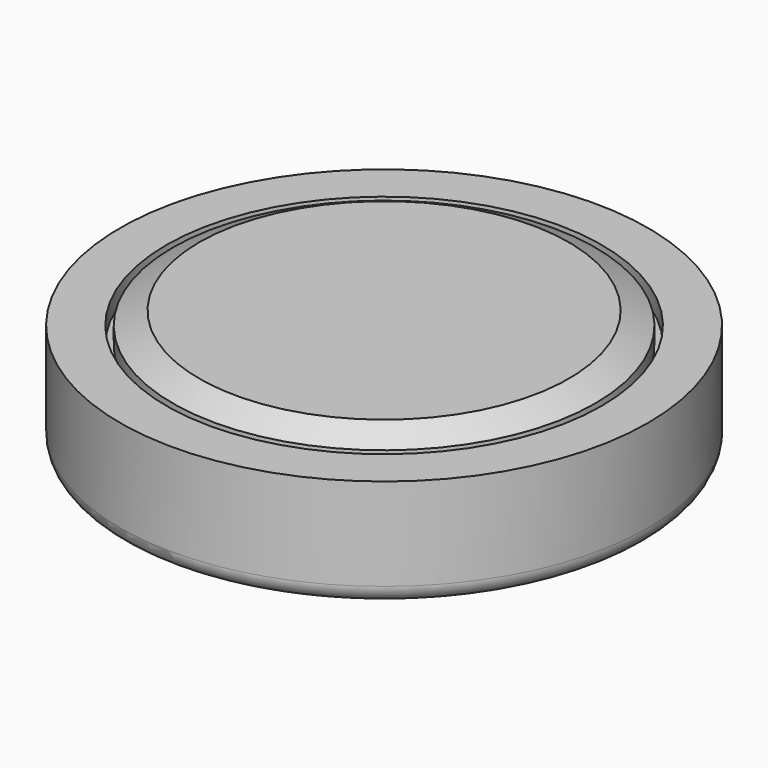
from build123d import *

# Parameters (mm, degrees)
F0_R      = 1.25
F1_DEPTH  = 3
F3_DEPTH  = 6
F4_R      = 1.2192
F5_DEPTH  = 7
F4_R_2    = 2
F4_R_3    = 0.9271
F7_R      = 24
F7_R_2    = 22
F7_R_3    = 21
F8_DEPTH  = 1.5
F9_DEPTH  = 2
F12_DEPTH = 2
F14_R     = 30
F14_R_2   = 24.75
F14_R_3   = 22.75
F14_R_4   = 2.75
F14_R_5   = 0.75
F14_R_6   = 1.875
F15_DEPTH = 2
F16_DEPTH = 1.5
F18_DEPTH = 8.5
F19_DEPTH = 10.5
F20_R     = 1.99999


# Not quite as in the source:
# - a fillet or chamfer that OpenCascade refuses, or shapes differently, is made with other operations: its cross-section is extruded or revolved along the edge and cut away or added
# - a fillet or chamfer is up to 0.001 mm smaller than in the source, because OpenCascade refuses the exact size


with BuildPart() as f1:
    # F0 (on Top) → F1 (new body)
    with BuildSketch(Plane.XY):
        with BuildLine():
            Line((8.25, 11.25), (8.25, 14.5))
            Line((8.25, 14.5), (-14.5, 14.5))
            Line((-14.5, 14.5), (-14.5, -8.25))
            Line((-14.5, -8.25), (-11.25, -8.25))
            ThreePointArc((-11.25, -8.25), (-9.1286796564, -9.1286796564), (-8.25, -11.25))
            Line((-8.25, -11.25), (-8.25, -14.5))
            Line((-8.25, -14.5), (14.5, -14.5))
            Line((14.5, -14.5), (14.5, 8.25))
            Line((14.5, 8.25), (11.25, 8.25))
            ThreePointArc((11.25, 8.25), (9.1286796564, 9.1286796564), (8.25, 11.25))
        make_face()
        with Locations((8.75, -11.75)):
            Circle(F0_R, mode=Mode.SUBTRACT)
        with Locations((-8.75, 11.75)):
            Circle(F0_R, mode=Mode.SUBTRACT)
    extrude(amount=-F1_DEPTH)

    # F2 (on Top) → F3 (join)
    with BuildSketch(Plane.XY):
        with BuildLine():
            ThreePointArc((7.5137790093, -9.675), (11.0024154817, -5.3860331941), (12.25, 0))
            ThreePointArc((12.25, 0), (11.0024154817, 5.3860331941), (7.5137790093, 9.675))
            Line((7.5137790093, 9.675), (-7.5137790093, 9.675))
            ThreePointArc((-7.5137790093, 9.675), (-12.25, 0), (-7.5137790093, -9.675))
            Line((-7.5137790093, -9.675), (7.5137790093, -9.675))
        make_face()
        with BuildLine():
            ThreePointArc((-7.5137790093, -9.675), (0, -12.25), (7.5137790093, -9.675))
            Line((7.5137790093, -9.675), (-7.5137790093, -9.675))
        make_face()
        with BuildLine():
            ThreePointArc((-7.5137790093, -9.675), (-12.25, 0), (-7.5137790093, 9.675))
            Line((-7.5137790093, 9.675), (-8.714591153, 9.675))
            Line((-8.714591153, 9.675), (-12.8, 7.175))
            Line((-12.8, 7.175), (-12.8, -5.5770184845))
            Line((-12.8, -5.5770184845), (-8.2916002721, -9.675))
            Line((-8.2916002721, -9.675), (-7.5137790093, -9.675))
        make_face()
        with BuildLine():
            ThreePointArc((7.5137790093, 9.675), (11.0024154817, 5.3860331941), (12.25, 0))
            ThreePointArc((12.25, 0), (11.0024154817, -5.3860331941), (7.5137790093, -9.675))
            Line((7.5137790093, -9.675), (7.8, -9.675))
            Line((7.8, -9.675), (12.8, -6.175))
            Line((12.8, -6.175), (12.8, 7.175))
            Line((12.8, 7.175), (8.17, 9.675))
            Line((8.17, 9.675), (7.5137790093, 9.675))
        make_face()
        with BuildLine():
            Line((-7.5137790093, 9.675), (7.5137790093, 9.675))
            ThreePointArc((7.5137790093, 9.675), (0, 12.25), (-7.5137790093, 9.675))
        make_face()
    extrude(amount=F3_DEPTH)


with BuildPart() as f5:
    # F4 (on Top) → F5 (new body)
    with BuildSketch(Plane.XY):
        with BuildLine():
            ThreePointArc((-9.1239573499, -12.75), (-8.9863719636, -12.2583896898), (-8.94, -11.75))
            ThreePointArc((-8.94, -11.75), (-8.9863719636, -11.2416103102), (-9.1239573499, -10.75))
            ThreePointArc((-9.1239573499, -10.75), (-9.7630299449, -9.7630299449), (-10.75, -9.1239573499))
            ThreePointArc((-10.75, -9.1239573499), (-11.75, -8.94), (-12.75, -9.1239573499))
            ThreePointArc((-12.75, -9.1239573499), (-13.7369700551, -13.7369700551), (-9.1239573499, -12.75))
        make_face()
        with Locations((-11.75, -11.75)):
            Circle(F4_R, mode=Mode.SUBTRACT)
        with BuildLine():
            ThreePointArc((-9.1239573499, -10.75), (-8.9863719636, -11.2416103102), (-8.94, -11.75))
            ThreePointArc((-8.94, -11.75), (-8.9863719636, -12.2583896898), (-9.1239573499, -12.75))
            Line((-9.1239573499, -12.75), (-8.75, -12.75))
            ThreePointArc((-8.75, -12.75), (-8.0428932188, -12.4571067812), (-7.75, -11.75))
            ThreePointArc((-7.75, -11.75), (-8.0428932188, -11.0428932188), (-8.75, -10.75))
            Line((-8.75, -10.75), (-9.1239573499, -10.75))
        make_face()
        with BuildLine():
            ThreePointArc((-12.75, -9.1239573499), (-11.75, -8.94), (-10.75, -9.1239573499))
            Line((-10.75, -9.1239573499), (-10.75, -8.75))
            ThreePointArc((-10.75, -8.75), (-11.0428932188, -8.0428932188), (-11.75, -7.75))
            ThreePointArc((-11.75, -7.75), (-12.4571067812, -8.0428932188), (-12.75, -8.75))
            Line((-12.75, -8.75), (-12.75, -9.1239573499))
        make_face()
    extrude(amount=F5_DEPTH)



with BuildPart() as f5b:
    # F4 (on Top) → F5, piece 2 (new body)
    with BuildSketch(Plane.XY):
        with Locations((8.75, -11.75)):
            Circle(F4_R_2)
        with Locations((8.75, -11.75)):
            Circle(F4_R_3, mode=Mode.SUBTRACT)
    extrude(amount=F5_DEPTH)


with BuildPart() as f5c:
    # F4 (on Top) → F5, piece 3 (new body)
    with BuildSketch(Plane.XY):
        with BuildLine():
            ThreePointArc((9.1239573499, 10.75), (8.94, 11.75), (9.1239573499, 12.75))
            Line((9.1239573499, 12.75), (8.75, 12.75))
            ThreePointArc((8.75, 12.75), (8.0428932188, 12.4571067812), (7.75, 11.75))
            ThreePointArc((7.75, 11.75), (8.0428932188, 11.0428932188), (8.75, 10.75))
            Line((8.75, 10.75), (9.1239573499, 10.75))
        make_face()
        with BuildLine():
            Line((12.75, 8.75), (12.75, 9.1239573499))
            ThreePointArc((12.75, 9.1239573499), (11.75, 8.94), (10.75, 9.1239573499))
            Line((10.75, 9.1239573499), (10.75, 8.75))
            ThreePointArc((10.75, 8.75), (11.0428932188, 8.0428932188), (11.75, 7.75))
            ThreePointArc((11.75, 7.75), (12.4571067812, 8.0428932188), (12.75, 8.75))
        make_face()
        with BuildLine():
            ThreePointArc((12.75, 9.1239573499), (14.0636659223, 10.1553056719), (14.56, 11.75))
            ThreePointArc((14.56, 11.75), (12.2583896898, 14.5136280364), (9.1239573499, 12.75))
            ThreePointArc((9.1239573499, 12.75), (8.94, 11.75), (9.1239573499, 10.75))
            ThreePointArc((9.1239573499, 10.75), (9.7630299449, 9.7630299449), (10.75, 9.1239573499))
            ThreePointArc((10.75, 9.1239573499), (11.75, 8.94), (12.75, 9.1239573499))
        make_face()
        with Locations((11.75, 11.75)):
            Circle(F4_R, mode=Mode.SUBTRACT)
    extrude(amount=F5_DEPTH)


with BuildPart() as f5d:
    # F4 (on Top) → F5, piece 4 (new body)
    with BuildSketch(Plane.XY):
        with Locations((-8.75, 11.75)):
            Circle(F4_R_2)
        with Locations((-8.75, 11.75)):
            Circle(F4_R_3, mode=Mode.SUBTRACT)
    extrude(amount=F5_DEPTH)


with BuildPart() as f5_1:
    add(f5.part)

    add(f5b.part)  # F8 merges F5b

    add(f5c.part)  # F8 merges F5c

    add(f5d.part)  # F8 merges F5d
    # F7 (on offset) → F8 (join)
    with BuildSketch(Plane.XY.offset(7)):
        Circle(F7_R)
        Circle(F7_R_2, mode=Mode.SUBTRACT)
        Circle(F7_R_2)
        Circle(F7_R_3, mode=Mode.SUBTRACT)
        Circle(F7_R_3)
    extrude(amount=F8_DEPTH)

    # F4 (on Top) → F9 (join)
    with BuildSketch(Plane.XY):
        with BuildLine():
            ThreePointArc((-9.1239573499, -12.75), (-8.9863719636, -12.2583896898), (-8.94, -11.75))
            ThreePointArc((-8.94, -11.75), (-8.9863719636, -11.2416103102), (-9.1239573499, -10.75))
            ThreePointArc((-9.1239573499, -10.75), (-9.7630299449, -9.7630299449), (-10.75, -9.1239573499))
            ThreePointArc((-10.75, -9.1239573499), (-11.75, -8.94), (-12.75, -9.1239573499))
            ThreePointArc((-12.75, -9.1239573499), (-13.7369700551, -13.7369700551), (-9.1239573499, -12.75))
        make_face()
        with Locations((-11.75, -11.75)):
            Circle(F4_R, mode=Mode.SUBTRACT)
        with BuildLine():
            ThreePointArc((12.75, 9.1239573499), (14.0636659223, 10.1553056719), (14.56, 11.75))
            ThreePointArc((14.56, 11.75), (12.2583896898, 14.5136280364), (9.1239573499, 12.75))
            ThreePointArc((9.1239573499, 12.75), (8.94, 11.75), (9.1239573499, 10.75))
            ThreePointArc((9.1239573499, 10.75), (9.7630299449, 9.7630299449), (10.75, 9.1239573499))
            ThreePointArc((10.75, 9.1239573499), (11.75, 8.94), (12.75, 9.1239573499))
        make_face()
        with Locations((11.75, 11.75)):
            Circle(F4_R, mode=Mode.SUBTRACT)
    extrude(amount=-F9_DEPTH)

    # F10 (on Front) → F11 (revolve, cut)
    with BuildSketch(Plane.XZ):
        Polygon((-24, 8.5), (-24, 7), (-21, 8.5), align=None)
    revolve(axis=Axis((0, 0, 4.2050974444), (0, 0, 1)), mode=Mode.SUBTRACT)

    # F7 (on offset) → F12 (join)
    with BuildSketch(Plane.XY.offset(7)):
        Circle(F7_R)
        Circle(F7_R_2, mode=Mode.SUBTRACT)
    extrude(amount=-F12_DEPTH)


with BuildPart() as f15:
    # F14 (on offset) → F15 (new body)
    with BuildSketch(Plane(origin=(0, 0, -3.5), x_dir=(1, 0, 0), z_dir=(0, 0, -1))):
        Circle(F14_R)
        Circle(F14_R_2, mode=Mode.SUBTRACT)
        Circle(F14_R_2)
        Circle(F14_R_3, mode=Mode.SUBTRACT)
        Circle(F14_R_3)
        with Locations((11.75, -11.75)):
            Circle(F14_R_4, mode=Mode.SUBTRACT)
        with Locations((-11.75, 11.75)):
            Circle(F14_R_4, mode=Mode.SUBTRACT)
        with Locations((1.5, 1.5)):
            Circle(F14_R_5, mode=Mode.SUBTRACT)
        with Locations((-11.75, 11.75)):
            Circle(F14_R_4)
        with Locations((-11.75, 11.75)):
            Circle(F14_R_6, mode=Mode.SUBTRACT)
        with Locations((11.75, -11.75)):
            Circle(F14_R_4)
        with Locations((11.75, -11.75)):
            Circle(F14_R_6, mode=Mode.SUBTRACT)
    extrude(amount=F15_DEPTH)

    # F14 (on offset) → F16 (join)
    with BuildSketch(Plane(origin=(0, 0, -3.5), x_dir=(1, 0, 0), z_dir=(0, 0, -1))):
        with Locations((11.75, -11.75)):
            Circle(F14_R_4)
        with Locations((11.75, -11.75)):
            Circle(F14_R_6, mode=Mode.SUBTRACT)
        with Locations((-11.75, 11.75)):
            Circle(F14_R_4)
        with Locations((-11.75, 11.75)):
            Circle(F14_R_6, mode=Mode.SUBTRACT)
    extrude(amount=-F16_DEPTH)

    # F17: chamfer of 2 on 2 edges, made by hand

    # F17_s1 → F17_t2 (revolve, cut)
    with BuildSketch(Plane.XZ.offset(11.75)):
        Polygon((-7.875, -5.5), (-9.875, -3.5), (-9.875, -5.5), align=None)
    revolve(axis=Axis((-11.75, -11.75, -5.5), (0, 0, -1)), mode=Mode.SUBTRACT)

    # F17_s3 → F17_t4 (revolve, cut)
    with BuildSketch(Plane.XZ.offset(-11.75)):
        Polygon((15.625, -5.5), (13.625, -3.5), (13.625, -5.5), align=None)
    revolve(axis=Axis((11.75, 11.75, -5.5), (0, 0, -1)), mode=Mode.SUBTRACT)

    # F14 (on offset) → F18 (join, through all)
    with BuildSketch(Plane(origin=(0, 0, -3.5), x_dir=(1, 0, 0), z_dir=(0, 0, -1))):
        Circle(F14_R_2)
        Circle(F14_R_3, mode=Mode.SUBTRACT)
    extrude(amount=-F18_DEPTH)

    # F14 (on offset) → F19 (join)
    with BuildSketch(Plane(origin=(0, 0, -3.5), x_dir=(1, 0, 0), z_dir=(0, 0, -1))):
        Circle(F14_R)
        Circle(F14_R_2, mode=Mode.SUBTRACT)
    extrude(amount=-F19_DEPTH)

    # F20 (radius 2 in the source; OpenCascade refuses exactly that, so slightly less here)
    f20_edges = [f15.edges().sort_by_distance(p)[0] for p in [
        (-30, 0, -5.5),
    ]]
    fillet(f20_edges, radius=F20_R)


solid = Compound([f1.part, f5_1.part, f15.part])
